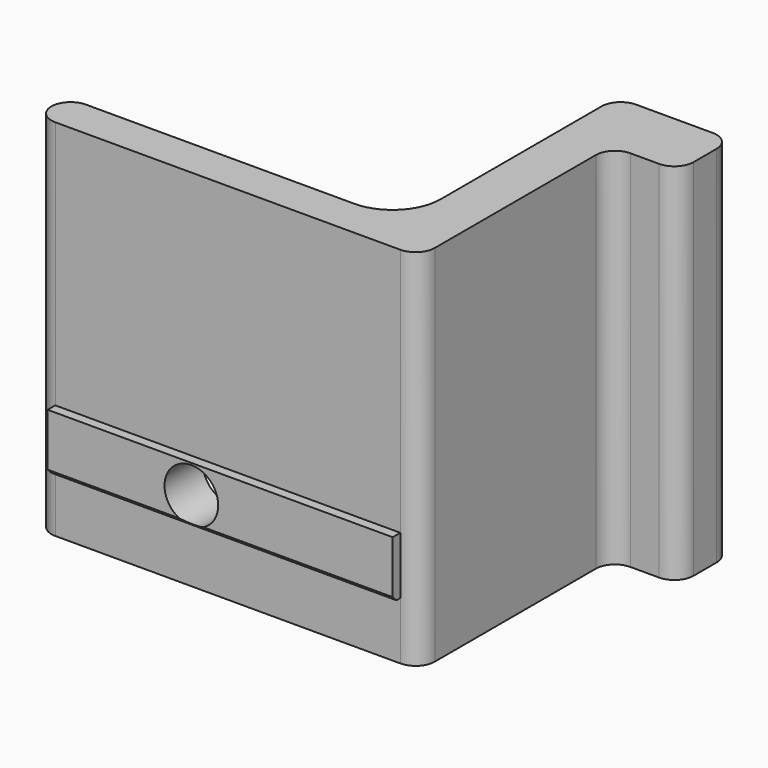
from build123d import *

# Parameters (mm, degrees)
F1_DEPTH    = 38
F2_W        = 36
F2_H        = 6
F2_R        = 2.8
F3_DEPTH    = 1
F4_DEPTH    = 4
F5_T1_DEPTH = 38.571682988


# Not quite as in the source:
# - a fillet or chamfer that OpenCascade refuses, or shapes differently, is made with other operations: its cross-section is extruded or revolved along the edge and cut away or added


with BuildPart() as f1:
    # F0 (on Top) → F1 (new body)
    with BuildSketch(Plane.XY):
        with BuildLine():
            ThreePointArc((0, 2), (0.5857864376, 0.5857864376), (2, 0))
            Line((2, 0), (38, 0))
            ThreePointArc((38, 0), (39.4142135624, 0.5857864376), (40, 2))
            Line((40, 2), (40, 23))
            ThreePointArc((40, 23), (40.5857864376, 24.4142135624), (42, 25))
            Line((42, 25), (45, 25))
            ThreePointArc((45, 25), (46.4142135624, 25.5857864376), (47, 27))
            Line((47, 27), (47, 30))
            ThreePointArc((47, 30), (46.4142135624, 31.4142135624), (45, 32))
            Line((45, 32), (40, 32))
            Line((40, 32), (37, 32))
            ThreePointArc((37, 32), (35.5857864376, 31.4142135624), (35, 30))
            Line((35, 30), (35, 9))
            ThreePointArc((35, 9), (33.5355339059, 5.4644660941), (30, 4))
            Line((30, 4), (2, 4))
            ThreePointArc((2, 4), (0.5857864376, 3.4142135624), (0, 2))
        make_face()
    extrude(amount=F1_DEPTH)

    # F2 (on face) → F3 (join)
    with BuildSketch(Plane.XZ):
        with Locations((20, 9)):
            Rectangle(F2_W, F2_H)
        with Locations((17, 9)):
            Circle(F2_R, mode=Mode.SUBTRACT)
    extrude(amount=F3_DEPTH)

    # F4 (cut): a face of the model
    f4_faces = [f1.faces().sort_by_distance(p)[0] for p in [
        (17, 0, 9),
    ]]
    extrude(f4_faces, amount=-F4_DEPTH, mode=Mode.SUBTRACT)

    # F5: chamfer of 0.5 on 1 edges, made by hand

    # F5_s2 → F5_t1 (cut)
    with BuildSketch(Plane.YZ.offset(0.714158506)):
        Polygon((-0.5, 6), (-1, 6.5), (-1, 6), align=None)
    extrude(amount=F5_T1_DEPTH, mode=Mode.SUBTRACT)


solid = f1.part
